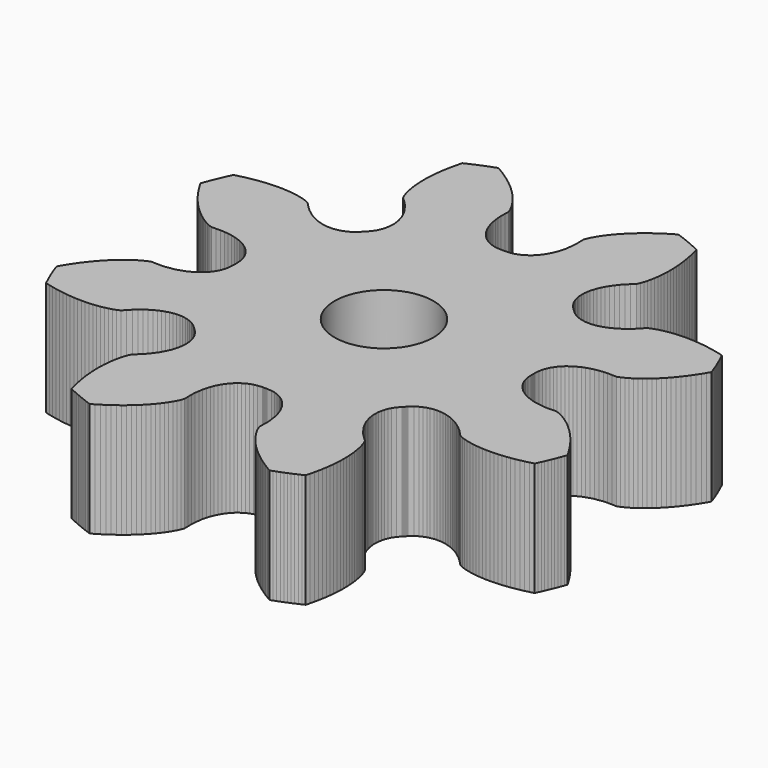
from build123d import *

# Parameters (mm, degrees)
F0_R     = 1.3
F1_DEPTH = 3


# Not quite as in the source:
# - ends of sketch curves that miss each other by under 0.0002 mm in the source are joined


with BuildPart() as f1:
    # F0 (on Top) → F1 (new body)
    with BuildSketch(Plane.XY):
        Polygon((3.91873, -0.01261), (3.91875, 0), (3.91873, 0.01261), (3.918669, 0.02522), (3.918567, 0.037829), (3.918425, 0.050438), (3.918243, 0.063047), (3.927022, 0.180894), (3.946465, 0.280905), (3.974611, 0.359921), (4.009085, 0.438851), (4.050739, 0.504778), (4.097447, 0.573512), (4.150796, 0.631412), (4.209027, 0.689888), (4.273539, 0.739418), (4.342741, 0.789047), (4.418306, 0.828977), (4.498112, 0.870334), (4.584187, 0.902056), (4.674962, 0.93187), (4.771145, 0.955731), (4.873257, 0.970539), (4.979177, 0.986368), (5.091067, 0.991698), (5.208217, 0.989239), (5.32907, 0.986364), (5.410163, 1.016651), (5.489651, 1.055105), (5.56805, 1.098614), (5.64541, 1.146577), (5.721741, 1.198614), (5.797032, 1.254457), (5.87126, 1.313903), (5.944393, 1.376794), (6.016393, 1.443001), (6.08722, 1.512416), (6.15683, 1.584946), (6.225176, 1.660508), (6.292211, 1.739031), (6.357886, 1.820446), (6.42215, 1.904693), (6.484952, 1.991715), (6.546241, 2.081459), (6.605965, 2.173872), (6.664072, 2.268905), (6.72051, 2.36651), (6.694499, 2.43912), (6.667703, 2.511445), (6.640127, 2.583475), (6.611771, 2.655203), (6.582642, 2.726619), (6.5527401565, 2.797716063), (6.5220715212, 2.8684861381), (6.4906377963, 2.9389182162), (6.4584439317, 3.0090073474), (6.4254934628, 3.0787429253), (6.3165686129, 3.1078523901), (6.2082822804, 3.1339630151), (6.100705176, 3.1570776287), (5.9939087176, 3.1771983522), (5.8879671512, 3.1943244784), (5.782954016, 3.2084545932), (5.6789456796, 3.219584454), (5.5760206307, 3.2277076967), (5.474262308, 3.2328101792), (5.3737541501, 3.234874931), (5.2745880809, 3.2338764962), (5.176860974, 3.2297802266), (5.0806774812, 3.222538039), (4.9861556894, 3.2120855865), (4.8934299487, 3.1983337739), (4.8026600654, 3.1811553217), (4.7140433223, 3.1603685037), (4.6278413488, 3.1356975481), (4.5444437608, 3.1066821284), (4.4656862075, 3.0707568613), (4.3822631637, 2.9832679535), (4.3011643799, 2.8986916185), (4.218277323, 2.8233423199), (4.1321877795, 2.7596383629), (4.0495128546, 2.6979051124), (3.9646289282, 2.6467657358), (3.8793596285, 2.6036597993), (3.796064571, 2.5652264244), (3.7103893921, 2.5380388758), (3.6287220944, 2.5128411257), (3.5446958885, 2.4990009246), (3.464056017, 2.4884070508), (3.3815317058, 2.488580292), (3.3028667835, 2.491798335), (3.2212369625, 2.5073730689), (3.1451657079, 2.5245366718), (3.0649769705, 2.5559718109), (2.9892019936, 2.5919423328), (2.9047352601, 2.648912512), (2.8151971569, 2.7260352344), (2.8064099409, 2.7350798372), (2.7975944407, 2.7440961558), (2.7887506561, 2.7530841901), (2.7798771732, 2.7620439401), (2.7709746988, 2.7709746988), (2.7620439401, 2.7798771732), (2.7530841901, 2.7887506561), (2.7440961558, 2.7975944407), (2.7350798372, 2.8064099409), (2.7260352344, 2.8151971569), (2.648912512, 2.9047352601), (2.5919423328, 2.9892019936), (2.5559718109, 3.0649769705), (2.5245366718, 3.1451657079), (2.5073730689, 3.2212369625), (2.491798335, 3.3028667835), (2.488580292, 3.3815317058), (2.4884070508, 3.464056017), (2.4990009246, 3.5446958885), (2.5128411257, 3.6287220944), (2.5380388758, 3.7103893921), (2.5652264244, 3.796064571), (2.6036597993, 3.8793596285), (2.6467657358, 3.9646289282), (2.6979051124, 4.0495128546), (2.7596383629, 4.1321877795), (2.8233423199, 4.218277323), (2.8986916185, 4.3011643799), (2.9832679535, 4.3822631637), (3.0707568613, 4.4656862075), (3.1066821284, 4.5444437608), (3.1356975481, 4.6278413488), (3.1603685037, 4.7140433223), (3.1811553217, 4.8026600654), (3.1983337739, 4.8934299487), (3.2120855865, 4.9861556894), (3.222538039, 5.0806774812), (3.2297802266, 5.176860974), (3.2338764962, 5.2745880809), (3.234874931, 5.3737541501), (3.2328101792, 5.474262308), (3.2277076967, 5.5760206307), (3.219584454, 5.6789456796), (3.2084545932, 5.782954016), (3.1943244784, 5.8879671512), (3.1771983522, 5.9939087176), (3.1570776287, 6.100705176), (3.1339630151, 6.2082822804), (3.1078523901, 6.3165686129), (3.0787429253, 6.4254934628), (3.0090073474, 6.4584439317), (2.9389182162, 6.4906377963), (2.8684861381, 6.5220715212), (2.797716063, 6.5527401565), (2.7266200117, 6.5826415809), (2.655203, 6.611771), (2.583475, 6.640127), (2.511445, 6.667703), (2.43912, 6.694499), (2.36651, 6.72051), (2.268905, 6.664072), (2.173872, 6.605965), (2.081459, 6.546241), (1.991715, 6.484952), (1.904693, 6.42215), (1.820446, 6.357886), (1.739031, 6.292211), (1.660508, 6.225176), (1.584946, 6.15683), (1.512416, 6.08722), (1.443001, 6.016393), (1.376794, 5.944393), (1.313903, 5.87126), (1.254457, 5.797032), (1.198614, 5.721741), (1.146577, 5.64541), (1.098614, 5.56805), (1.055105, 5.489651), (1.016651, 5.410163), (0.986364, 5.32907), (0.989239, 5.208217), (0.991698, 5.091067), (0.986368, 4.979177), (0.970539, 4.873257), (0.955731, 4.771145), (0.93187, 4.674962), (0.902056, 4.584187), (0.870334, 4.498112), (0.828977, 4.418306), (0.789047, 4.342741), (0.739418, 4.273539), (0.689888, 4.209027), (0.631412, 4.150796), (0.573512, 4.097447), (0.504778, 4.050739), (0.438851, 4.009085), (0.359921, 3.974611), (0.280905, 3.946465), (0.180894, 3.927022), (0.063047, 3.918243), (0.050438, 3.918425), (0.037829, 3.918567), (0.02522, 3.918669), (0.01261, 3.91873), (0, 3.91875), (-0.01261, 3.91873), (-0.02522, 3.918669), (-0.037829, 3.918567), (-0.050438, 3.918425), (-0.063047, 3.918243), (-0.180894, 3.927022), (-0.280905, 3.946465), (-0.359921, 3.974611), (-0.438851, 4.009085), (-0.504778, 4.050739), (-0.573512, 4.097447), (-0.631412, 4.150796), (-0.689888, 4.209027), (-0.739418, 4.273539), (-0.789047, 4.342741), (-0.828977, 4.418306), (-0.870334, 4.498112), (-0.902056, 4.584187), (-0.93187, 4.674962), (-0.955731, 4.771145), (-0.970539, 4.873257), (-0.986368, 4.979177), (-0.991698, 5.091067), (-0.989239, 5.208217), (-0.986364, 5.32907), (-1.016651, 5.410163), (-1.055105, 5.489651), (-1.098614, 5.56805), (-1.146577, 5.64541), (-1.198614, 5.721741), (-1.254457, 5.797032), (-1.313903, 5.87126), (-1.376794, 5.944393), (-1.443001, 6.016393), (-1.512416, 6.08722), (-1.584946, 6.15683), (-1.660508, 6.225176), (-1.739031, 6.292211), (-1.820446, 6.357886), (-1.904693, 6.42215), (-1.991715, 6.484952), (-2.081459, 6.546241), (-2.173872, 6.605965), (-2.268905, 6.664072), (-2.36651, 6.72051), (-2.43912, 6.694499), (-2.511445, 6.667703), (-2.583475, 6.640127), (-2.655203, 6.611771), (-2.726619, 6.582642), (-2.797716063, 6.5527401565), (-2.8684861381, 6.5220715212), (-2.9389182162, 6.4906377963), (-3.0090073474, 6.4584439317), (-3.0787429253, 6.4254934628), (-3.1078523901, 6.3165686129), (-3.1339630151, 6.2082822804), (-3.1570776287, 6.100705176), (-3.1771983522, 5.9939087176), (-3.1943244784, 5.8879671512), (-3.2084545932, 5.782954016), (-3.219584454, 5.6789456796), (-3.2277076967, 5.5760206307), (-3.2328101792, 5.474262308), (-3.234874931, 5.3737541501), (-3.2338764962, 5.2745880809), (-3.2297802266, 5.176860974), (-3.222538039, 5.0806774812), (-3.2120855865, 4.9861556894), (-3.1983337739, 4.8934299487), (-3.1811553217, 4.8026600654), (-3.1603685037, 4.7140433223), (-3.1356975481, 4.6278413488), (-3.1066821284, 4.5444437608), (-3.0707568613, 4.4656862075), (-2.9832679535, 4.3822631637), (-2.8986916185, 4.3011643799), (-2.8233423199, 4.218277323), (-2.7596383629, 4.1321877795), (-2.6979051124, 4.0495128546), (-2.6467657358, 3.9646289282), (-2.6036597993, 3.8793596285), (-2.5652264244, 3.796064571), (-2.5380388758, 3.7103893921), (-2.5128411257, 3.6287220944), (-2.4990009246, 3.5446958885), (-2.4884070508, 3.464056017), (-2.488580292, 3.3815317058), (-2.491798335, 3.3028667835), (-2.5073730689, 3.2212369625), (-2.5245366718, 3.1451657079), (-2.5559718109, 3.0649769705), (-2.5919423328, 2.9892019936), (-2.648912512, 2.9047352601), (-2.7260352344, 2.8151971569), (-2.7350798372, 2.8064099409), (-2.7440961558, 2.7975944407), (-2.7530841901, 2.7887506561), (-2.7620439401, 2.7798771732), (-2.7709746988, 2.7709746988), (-2.7798771732, 2.7620439401), (-2.7887506561, 2.7530841901), (-2.7975944407, 2.7440961558), (-2.8064099409, 2.7350798372), (-2.8151971569, 2.7260352344), (-2.9047352601, 2.648912512), (-2.9892019936, 2.5919423328), (-3.0649769705, 2.5559718109), (-3.1451657079, 2.5245366718), (-3.2212369625, 2.5073730689), (-3.3028667835, 2.491798335), (-3.3815317058, 2.488580292), (-3.464056017, 2.4884070508), (-3.5446958885, 2.4990009246), (-3.6287220944, 2.5128411257), (-3.7103893921, 2.5380388758), (-3.796064571, 2.5652264244), (-3.8793596285, 2.6036597993), (-3.9646289282, 2.6467657358), (-4.0495128546, 2.6979051124), (-4.1321877795, 2.7596383629), (-4.218277323, 2.8233423199), (-4.3011643799, 2.8986916185), (-4.3822631637, 2.9832679535), (-4.4656862075, 3.0707568613), (-4.5444437608, 3.1066821284), (-4.6278413488, 3.1356975481), (-4.7140433223, 3.1603685037), (-4.8026600654, 3.1811553217), (-4.8934299487, 3.1983337739), (-4.9861556894, 3.2120855865), (-5.0806774812, 3.222538039), (-5.176860974, 3.2297802266), (-5.2745880809, 3.2338764962), (-5.3737541501, 3.234874931), (-5.474262308, 3.2328101792), (-5.5760206307, 3.2277076967), (-5.6789456796, 3.219584454), (-5.782954016, 3.2084545932), (-5.8879671512, 3.1943244784), (-5.9939087176, 3.1771983522), (-6.100705176, 3.1570776287), (-6.2082822804, 3.1339630151), (-6.3165686129, 3.1078523901), (-6.4254934628, 3.0787429253), (-6.4584439317, 3.0090073474), (-6.4906377963, 2.9389182162), (-6.5220715212, 2.8684861381), (-6.5527401565, 2.797716063), (-6.5826415809, 2.7266200117), (-6.611771, 2.655203), (-6.640127, 2.583475), (-6.667703, 2.511445), (-6.694499, 2.43912), (-6.72051, 2.36651), (-6.664072, 2.268905), (-6.605965, 2.173872), (-6.546241, 2.081459), (-6.484952, 1.991715), (-6.42215, 1.904693), (-6.357886, 1.820446), (-6.292211, 1.739031), (-6.225176, 1.660508), (-6.15683, 1.584946), (-6.08722, 1.512416), (-6.016393, 1.443001), (-5.944393, 1.376794), (-5.87126, 1.313903), (-5.797032, 1.254457), (-5.721741, 1.198614), (-5.64541, 1.146577), (-5.56805, 1.098614), (-5.489651, 1.055105), (-5.410163, 1.016651), (-5.32907, 0.986364), (-5.208217, 0.989239), (-5.091067, 0.991698), (-4.979177, 0.986368), (-4.873257, 0.970539), (-4.771145, 0.955731), (-4.674962, 0.93187), (-4.584187, 0.902056), (-4.498112, 0.870334), (-4.418306, 0.828977), (-4.342741, 0.789047), (-4.273539, 0.739418), (-4.209027, 0.689888), (-4.150796, 0.631412), (-4.097447, 0.573512), (-4.050739, 0.504778), (-4.009085, 0.438851), (-3.974611, 0.359921), (-3.946465, 0.280905), (-3.927022, 0.180894), (-3.918243, 0.063047), (-3.918425, 0.050438), (-3.918567, 0.037829), (-3.918669, 0.02522), (-3.91873, 0.01261), (-3.91875, 0), (-3.91873, -0.01261), (-3.918669, -0.02522), (-3.918567, -0.037829), (-3.918425, -0.050438), (-3.918243, -0.063047), (-3.927022, -0.180894), (-3.946465, -0.280905), (-3.974611, -0.359921), (-4.009085, -0.438851), (-4.050739, -0.504778), (-4.097447, -0.573512), (-4.150796, -0.631412), (-4.209027, -0.689888), (-4.273539, -0.739418), (-4.342741, -0.789047), (-4.418306, -0.828977), (-4.498112, -0.870334), (-4.584187, -0.902056), (-4.674962, -0.93187), (-4.771145, -0.955731), (-4.873257, -0.970539), (-4.979177, -0.986368), (-5.091067, -0.991698), (-5.208217, -0.989239), (-5.32907, -0.986364), (-5.410163, -1.016651), (-5.489651, -1.055105), (-5.56805, -1.098614), (-5.64541, -1.146577), (-5.721741, -1.198614), (-5.797032, -1.254457), (-5.87126, -1.313903), (-5.944393, -1.376794), (-6.016393, -1.443001), (-6.08722, -1.512416), (-6.15683, -1.584946), (-6.225176, -1.660508), (-6.292211, -1.739031), (-6.357886, -1.820446), (-6.42215, -1.904693), (-6.484952, -1.991715), (-6.546241, -2.081459), (-6.605965, -2.173872), (-6.664072, -2.268905), (-6.72051, -2.36651), (-6.694499, -2.43912), (-6.667703, -2.511445), (-6.640127, -2.583475), (-6.611771, -2.655203), (-6.582642, -2.726619), (-6.5527401565, -2.797716063), (-6.5220715212, -2.8684861381), (-6.4906377963, -2.9389182162), (-6.4584439317, -3.0090073474), (-6.4254934628, -3.0787429253), (-6.3165686129, -3.1078523901), (-6.2082822804, -3.1339630151), (-6.100705176, -3.1570776287), (-5.9939087176, -3.1771983522), (-5.8879671512, -3.1943244784), (-5.782954016, -3.2084545932), (-5.6789456796, -3.219584454), (-5.5760206307, -3.2277076967), (-5.474262308, -3.2328101792), (-5.3737541501, -3.234874931), (-5.2745880809, -3.2338764962), (-5.176860974, -3.2297802266), (-5.0806774812, -3.222538039), (-4.9861556894, -3.2120855865), (-4.8934299487, -3.1983337739), (-4.8026600654, -3.1811553217), (-4.7140433223, -3.1603685037), (-4.6278413488, -3.1356975481), (-4.5444437608, -3.1066821284), (-4.4656862075, -3.0707568613), (-4.3822631637, -2.9832679535), (-4.3011643799, -2.8986916185), (-4.218277323, -2.8233423199), (-4.1321877795, -2.7596383629), (-4.0495128546, -2.6979051124), (-3.9646289282, -2.6467657358), (-3.8793596285, -2.6036597993), (-3.796064571, -2.5652264244), (-3.7103893921, -2.5380388758), (-3.6287220944, -2.5128411257), (-3.5446958885, -2.4990009246), (-3.464056017, -2.4884070508), (-3.3815317058, -2.488580292), (-3.3028667835, -2.491798335), (-3.2212369625, -2.5073730689), (-3.1451657079, -2.5245366718), (-3.0649769705, -2.5559718109), (-2.9892019936, -2.5919423328), (-2.9047352601, -2.648912512), (-2.8151971569, -2.7260352344), (-2.8064099409, -2.7350798372), (-2.7975944407, -2.7440961558), (-2.7887506561, -2.7530841901), (-2.7798771732, -2.7620439401), (-2.7709746988, -2.7709746988), (-2.7620439401, -2.7798771732), (-2.7530841901, -2.7887506561), (-2.7440961558, -2.7975944407), (-2.7350798372, -2.8064099409), (-2.7260352344, -2.8151971569), (-2.648912512, -2.9047352601), (-2.5919423328, -2.9892019936), (-2.5559718109, -3.0649769705), (-2.5245366718, -3.1451657079), (-2.5073730689, -3.2212369625), (-2.491798335, -3.3028667835), (-2.488580292, -3.3815317058), (-2.4884070508, -3.464056017), (-2.4990009246, -3.5446958885), (-2.5128411257, -3.6287220944), (-2.5380388758, -3.7103893921), (-2.5652264244, -3.796064571), (-2.6036597993, -3.8793596285), (-2.6467657358, -3.9646289282), (-2.6979051124, -4.0495128546), (-2.7596383629, -4.1321877795), (-2.8233423199, -4.218277323), (-2.8986916185, -4.3011643799), (-2.9832679535, -4.3822631637), (-3.0707568613, -4.4656862075), (-3.1066821284, -4.5444437608), (-3.1356975481, -4.6278413488), (-3.1603685037, -4.7140433223), (-3.1811553217, -4.8026600654), (-3.1983337739, -4.8934299487), (-3.2120855865, -4.9861556894), (-3.222538039, -5.0806774812), (-3.2297802266, -5.176860974), (-3.2338764962, -5.2745880809), (-3.234874931, -5.3737541501), (-3.2328101792, -5.474262308), (-3.2277076967, -5.5760206307), (-3.219584454, -5.6789456796), (-3.2084545932, -5.782954016), (-3.1943244784, -5.8879671512), (-3.1771983522, -5.9939087176), (-3.1570776287, -6.100705176), (-3.1339630151, -6.2082822804), (-3.1078523901, -6.3165686129), (-3.0787429253, -6.4254934628), (-3.0090073474, -6.4584439317), (-2.9389182162, -6.4906377963), (-2.8684861381, -6.5220715212), (-2.797716063, -6.5527401565), (-2.7266200117, -6.5826415809), (-2.655203, -6.611771), (-2.583475, -6.640127), (-2.511445, -6.667703), (-2.43912, -6.694499), (-2.36651, -6.72051), (-2.268905, -6.664072), (-2.173872, -6.605965), (-2.081459, -6.546241), (-1.991715, -6.484952), (-1.904693, -6.42215), (-1.820446, -6.357886), (-1.739031, -6.292211), (-1.660508, -6.225176), (-1.584946, -6.15683), (-1.512416, -6.08722), (-1.443001, -6.016393), (-1.376794, -5.944393), (-1.313903, -5.87126), (-1.254457, -5.797032), (-1.198614, -5.721741), (-1.146577, -5.64541), (-1.098614, -5.56805), (-1.055105, -5.489651), (-1.016651, -5.410163), (-0.986364, -5.32907), (-0.989239, -5.208217), (-0.991698, -5.091067), (-0.986368, -4.979177), (-0.970539, -4.873257), (-0.955731, -4.771145), (-0.93187, -4.674962), (-0.902056, -4.584187), (-0.870334, -4.498112), (-0.828977, -4.418306), (-0.789047, -4.342741), (-0.739418, -4.273539), (-0.689888, -4.209027), (-0.631412, -4.150796), (-0.573512, -4.097447), (-0.504778, -4.050739), (-0.438851, -4.009085), (-0.359921, -3.974611), (-0.280905, -3.946465), (-0.180894, -3.927022), (-0.063047, -3.918243), (-0.050438, -3.918425), (-0.037829, -3.918567), (-0.02522, -3.918669), (-0.01261, -3.91873), (0, -3.91875), (0.01261, -3.91873), (0.02522, -3.918669), (0.037829, -3.918567), (0.050438, -3.918425), (0.063047, -3.918243), (0.180894, -3.927022), (0.280905, -3.946465), (0.359921, -3.974611), (0.438851, -4.009085), (0.504778, -4.050739), (0.573512, -4.097447), (0.631412, -4.150796), (0.689888, -4.209027), (0.739418, -4.273539), (0.789047, -4.342741), (0.828977, -4.418306), (0.870334, -4.498112), (0.902056, -4.584187), (0.93187, -4.674962), (0.955731, -4.771145), (0.970539, -4.873257), (0.986368, -4.979177), (0.991698, -5.091067), (0.989239, -5.208217), (0.986364, -5.32907), (1.016651, -5.410163), (1.055105, -5.489651), (1.098614, -5.56805), (1.146577, -5.64541), (1.198614, -5.721741), (1.254457, -5.797032), (1.313903, -5.87126), (1.376794, -5.944393), (1.443001, -6.016393), (1.512416, -6.08722), (1.584946, -6.15683), (1.660508, -6.225176), (1.739031, -6.292211), (1.820446, -6.357886), (1.904693, -6.42215), (1.991715, -6.484952), (2.081459, -6.546241), (2.173872, -6.605965), (2.268905, -6.664072), (2.36651, -6.72051), (2.43912, -6.694499), (2.511445, -6.667703), (2.583475, -6.640127), (2.655203, -6.611771), (2.726619, -6.582642), (2.797716063, -6.5527401565), (2.8684861381, -6.5220715212), (2.9389182162, -6.4906377963), (3.0090073474, -6.4584439317), (3.0787429253, -6.4254934628), (3.1078523901, -6.3165686129), (3.1339630151, -6.2082822804), (3.1570776287, -6.100705176), (3.1771983522, -5.9939087176), (3.1943244784, -5.8879671512), (3.2084545932, -5.782954016), (3.219584454, -5.6789456796), (3.2277076967, -5.5760206307), (3.2328101792, -5.474262308), (3.234874931, -5.3737541501), (3.2338764962, -5.2745880809), (3.2297802266, -5.176860974), (3.222538039, -5.0806774812), (3.2120855865, -4.9861556894), (3.1983337739, -4.8934299487), (3.1811553217, -4.8026600654), (3.1603685037, -4.7140433223), (3.1356975481, -4.6278413488), (3.1066821284, -4.5444437608), (3.0707568613, -4.4656862075), (2.9832679535, -4.3822631637), (2.8986916185, -4.3011643799), (2.8233423199, -4.218277323), (2.7596383629, -4.1321877795), (2.6979051124, -4.0495128546), (2.6467657358, -3.9646289282), (2.6036597993, -3.8793596285), (2.5652264244, -3.796064571), (2.5380388758, -3.7103893921), (2.5128411257, -3.6287220944), (2.4990009246, -3.5446958885), (2.4884070508, -3.464056017), (2.488580292, -3.3815317058), (2.491798335, -3.3028667835), (2.5073730689, -3.2212369625), (2.5245366718, -3.1451657079), (2.5559718109, -3.0649769705), (2.5919423328, -2.9892019936), (2.648912512, -2.9047352601), (2.7260352344, -2.8151971569), (2.7350798372, -2.8064099409), (2.7440961558, -2.7975944407), (2.7530841901, -2.7887506561), (2.7620439401, -2.7798771732), (2.7709746988, -2.7709746988), (2.7798771732, -2.7620439401), (2.7887506561, -2.7530841901), (2.7975944407, -2.7440961558), (2.8064099409, -2.7350798372), (2.8151971569, -2.7260352344), (2.9047352601, -2.648912512), (2.9892019936, -2.5919423328), (3.0649769705, -2.5559718109), (3.1451657079, -2.5245366718), (3.2212369625, -2.5073730689), (3.3028667835, -2.491798335), (3.3815317058, -2.488580292), (3.464056017, -2.4884070508), (3.5446958885, -2.4990009246), (3.6287220944, -2.5128411257), (3.7103893921, -2.5380388758), (3.796064571, -2.5652264244), (3.8793596285, -2.6036597993), (3.9646289282, -2.6467657358), (4.0495128546, -2.6979051124), (4.1321877795, -2.7596383629), (4.218277323, -2.8233423199), (4.3011643799, -2.8986916185), (4.3822631637, -2.9832679535), (4.4656862075, -3.0707568613), (4.5444437608, -3.1066821284), (4.6278413488, -3.1356975481), (4.7140433223, -3.1603685037), (4.8026600654, -3.1811553217), (4.8934299487, -3.1983337739), (4.9861556894, -3.2120855865), (5.0806774812, -3.222538039), (5.176860974, -3.2297802266), (5.2745880809, -3.2338764962), (5.3737541501, -3.234874931), (5.474262308, -3.2328101792), (5.5760206307, -3.2277076967), (5.6789456796, -3.219584454), (5.782954016, -3.2084545932), (5.8879671512, -3.1943244784), (5.9939087176, -3.1771983522), (6.100705176, -3.1570776287), (6.2082822804, -3.1339630151), (6.3165686129, -3.1078523901), (6.4254934628, -3.0787429253), (6.4584439317, -3.0090073474), (6.4906377963, -2.9389182162), (6.5220715212, -2.8684861381), (6.5527401565, -2.797716063), (6.5826415809, -2.7266200117), (6.611771, -2.655203), (6.640127, -2.583475), (6.667703, -2.511445), (6.694499, -2.43912), (6.72051, -2.36651), (6.664072, -2.268905), (6.605965, -2.173872), (6.546241, -2.081459), (6.484952, -1.991715), (6.42215, -1.904693), (6.357886, -1.820446), (6.292211, -1.739031), (6.225176, -1.660508), (6.15683, -1.584946), (6.08722, -1.512416), (6.016393, -1.443001), (5.944393, -1.376794), (5.87126, -1.313903), (5.797032, -1.254457), (5.721741, -1.198614), (5.64541, -1.146577), (5.56805, -1.098614), (5.489651, -1.055105), (5.410163, -1.016651), (5.32907, -0.986364), (5.208217, -0.989239), (5.091067, -0.991698), (4.979177, -0.986368), (4.873257, -0.970539), (4.771145, -0.955731), (4.674962, -0.93187), (4.584187, -0.902056), (4.498112, -0.870334), (4.418306, -0.828977), (4.342741, -0.789047), (4.273539, -0.739418), (4.209027, -0.689888), (4.150796, -0.631412), (4.097447, -0.573512), (4.050739, -0.504778), (4.009085, -0.438851), (3.974611, -0.359921), (3.946465, -0.280905), (3.927022, -0.180894), (3.918243, -0.063047), (3.918425, -0.050438), (3.918567, -0.037829), (3.918669, -0.02522), align=None)
        Circle(F0_R, mode=Mode.SUBTRACT)
    extrude(amount=F1_DEPTH)


solid = f1.part
